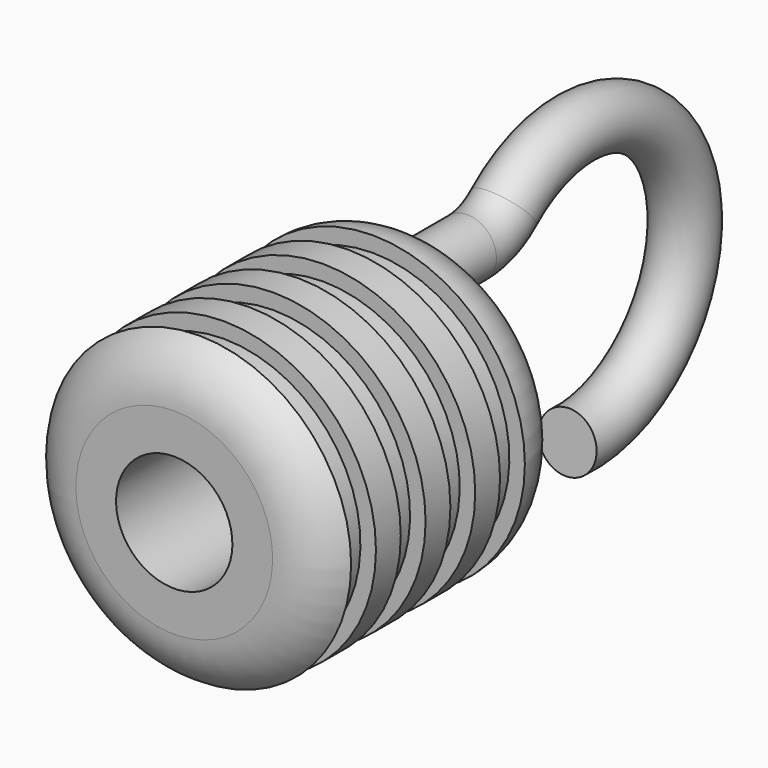
from build123d import *

# Parameters (mm, degrees)
F2_R        = 2.38125
F5_S5_R     = 2.38125
F5_T6_DEPTH = 21


# Not quite as in the source:
# - a fillet or chamfer that OpenCascade refuses, or shapes differently, is made with other operations: its cross-section is extruded or revolved along the edge and cut away or added


with BuildPart() as f1:
    # F0 (on Right) → F1 (revolve)
    with BuildSketch(Plane.YZ):
        Polygon((1.2978891239, 12.4533368552), (1.2978891239, 4.7625), (26.6978891239, 4.7625), (26.6978891239, 12.4533368552), (21.6178891239, 12.4533368552), (21.6178891239, 11.1833368552), (19.0778891239, 11.1833368552), (19.0778891239, 12.4533368552), (16.5378891239, 12.4533368552), (16.5378891239, 11.1833368552), (13.9978891239, 11.1833368552), (13.9978891239, 12.4533368552), (11.4578891239, 12.4533368552), (11.4578891239, 11.1833368552), (8.9178891239, 11.1833368552), (8.9178891239, 12.4533368552), (6.3778891239, 12.4533368552), (6.3778891239, 11.1833368552), (3.8378891239, 11.1833368552), (3.8378891239, 12.4533368552), align=None)
    revolve(axis=Axis((0, 14.6730239503, 0), (0, -1, 0)))

    # F4: sweep along a path in F3
    with BuildLine(Plane.YZ) as f4_path:
        ThreePointArc((41.5942855179, -9.9446065724), (52.3851323155, 3.8958588473), (35.4612426397, 8.5415897783))
        ThreePointArc((35.4612426397, 8.5415897783), (33.5207988127, 7.3890018952), (31.2997828747, 6.9879167713))
        Line((31.2997828747, 6.9879167713), (26.6969297081, 6.9879167713))
    # F2 (on face) → F4 (sweep)
    with BuildSketch(Plane(origin=(0, 26.6978891239, 0), x_dir=(-1, 0, 0), z_dir=(0, 1, 0))):
        with Locations((0, 7.62)):
            Circle(F2_R)
    sweep(path=f4_path.line)

    # F5: fillet of radius 5.08 on 2 edges, made by hand


with BuildPart() as f5_tool2:
    # F5_s3 → F5_t4 (revolve)
    with BuildSketch(Plane.YZ):
        with BuildLine():
            ThreePointArc((26.6978891239, 7.3733368552), (25.2099915723, 10.9654393036), (21.6178891239, 12.4533368552))
            Line((21.6178891239, 12.4533368552), (26.6978891239, 12.4533368552))
            Line((26.6978891239, 12.4533368552), (26.6978891239, 7.3733368552))
        make_face()
    revolve(axis=Axis((0, 26.6978891239, 0), (0, -1, 0)))

    # F5_s5 → F5_t6 (cut, symmetric)
    with BuildSketch(Plane.XZ.offset(-22.4)):
        with Locations((0, 7.62)):
            Circle(F5_S5_R)
    extrude(amount=F5_T6_DEPTH, both=True, mode=Mode.SUBTRACT)


with BuildPart() as f1_1:
    add(f1.part)

    # F5_t1: cut F5_tool2
    add(f5_tool2.part, mode=Mode.SUBTRACT)

    # F5_s7 → F5_t8 (revolve, cut)
    with BuildSketch(Plane.YZ):
        with BuildLine():
            ThreePointArc((3.8378891239, 12.4533368552), (1.9784800726, 10.5939278039), (1.2978891239, 8.0539278039))
            Line((1.2978891239, 8.0539278039), (1.2978891239, 12.4533368552))
            Line((1.2978891239, 12.4533368552), (3.8378891239, 12.4533368552))
        make_face()
    revolve(axis=Axis((0, 1.2978891239, 0), (0, -1, 0)), mode=Mode.SUBTRACT)


solid = f1_1.part
